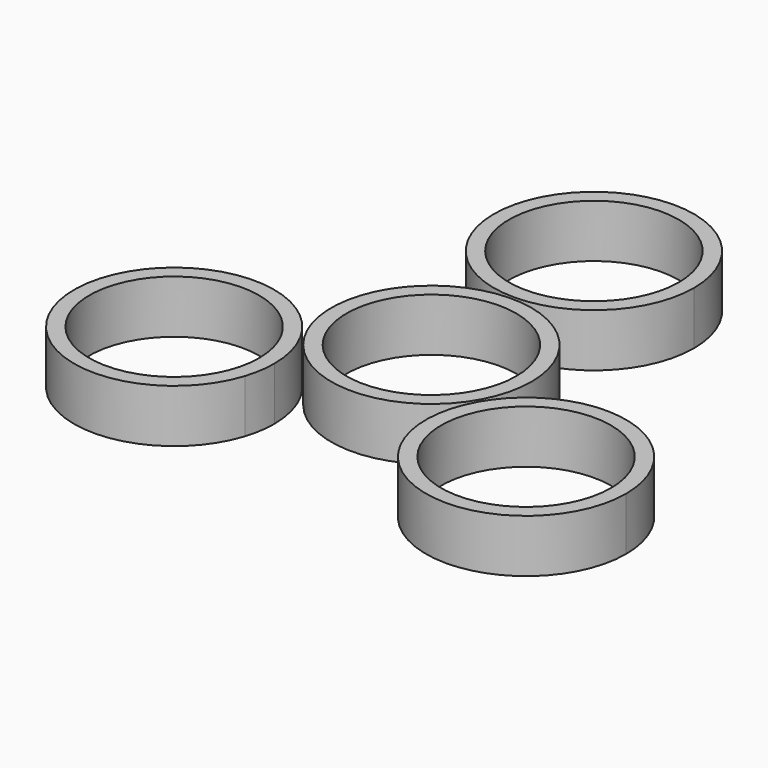
from build123d import *

# Parameters (mm, degrees)
F0_R     = 13.2
F0_R_2   = 11.2
F1_DEPTH = 7


# Not quite as in the source:
# - the program builds the solid bodies; features that only make, move or delete a surface that nothing else refers to are left out


with BuildPart() as f1:
    # F0 (on Top) → F1 (new body)
    with BuildSketch(Plane.XY):
        Circle(F0_R)
        Circle(F0_R_2, mode=Mode.SUBTRACT)
    extrude(amount=F1_DEPTH)


with BuildPart() as f1b:
    # F0 (on Top) → F1, piece 2 (new body)
    with BuildSketch(Plane.XY):
        with BuildLine():
            ThreePointArc((-9.7925592787, 17.9414493505), (4.7422683139, 14.4740434947), (13.2, 26.7927646637))
            ThreePointArc((13.2, 26.7927646637), (-4.7422683139, 39.1114858327), (-9.7925592787, 17.9414493505))
        make_face()
        with Locations((0, 26.7927646637)):
            Circle(F0_R_2, mode=Mode.SUBTRACT)
    extrude(amount=F1_DEPTH)


with BuildPart() as f1c:
    # F0 (on Top) → F1, piece 3 (new body)
    with BuildSketch(Plane.XY):
        with BuildLine():
            ThreePointArc((-10.6414712789, -17.4513297787), (-10.163755205, -15.448818085), (-10.0032148364, -13.3963823318))
            ThreePointArc((-10.0032148364, -13.3963823318), (-36.2426744678, -11.3439465787), (-10.6414712789, -17.4513297787))
        make_face()
        with Locations((-23.2032148364, -13.3963823318)):
            Circle(F0_R_2, mode=Mode.SUBTRACT)
    extrude(amount=F1_DEPTH)


with BuildPart() as f1d:
    # F0 (on Top) → F1, piece 4 (new body)
    with BuildSketch(Plane.XY):
        with BuildLine():
            ThreePointArc((20.4340305576, -0.4901195718), (14.9060235188, -23.6626677477), (36.4032148364, -13.3963823318))
            ThreePointArc((36.4032148364, -13.3963823318), (31.5004061539, -3.130096916), (20.4340305576, -0.4901195718))
        make_face()
        with Locations((23.2032148364, -13.3963823318)):
            Circle(F0_R_2, mode=Mode.SUBTRACT)
    extrude(amount=F1_DEPTH)


solid = Compound([f1.part, f1b.part, f1c.part, f1d.part])
